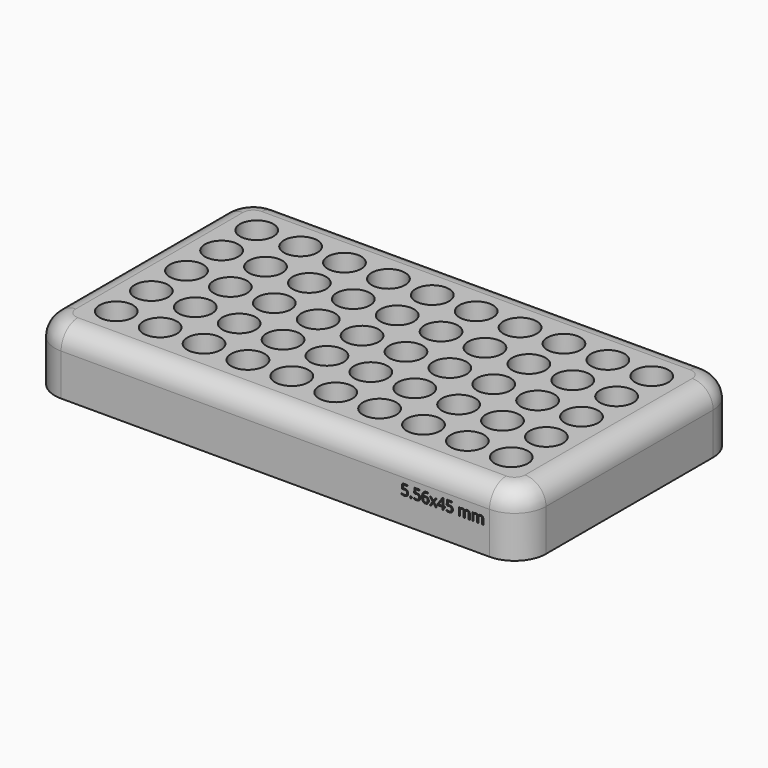
from build123d import *

# Parameters (mm, degrees)
F1_DEPTH     = 19.05
F2_R         = 6.35
F3_R         = 5.08
F4_DEPTH     = 9.525
F5_R         = 3.302
F6_DEPTH     = 15.24
F7_TEXT_SIZE = 4.4154715341
F8_DEPTH     = 1.5875


# Not quite as in the source:
# - Text() gives the source's letters only with a copy of the font that has no kerning and outlines rounded to 1/6400 em; it was checked with that copy


with BuildPart() as f1:
    # F0 (on Top) → F1 (new body)
    with BuildSketch(Plane.XY):
        with BuildLine():
            Line((96.05817945, 87.4035315238), (-34.11682055, 87.4035315238))
            ThreePointArc((-34.11682055, 87.4035315238), (-40.8520126408, 84.6137236146), (-43.64182055, 77.8785315238))
            Line((-43.64182055, 77.8785315238), (-43.64182055, 14.3785315238))
            ThreePointArc((-43.64182055, 14.3785315238), (-40.8520126408, 7.643339433), (-34.11682055, 4.8535315238))
            Line((-34.11682055, 4.8535315238), (96.05817945, 4.8535315238))
            ThreePointArc((96.05817945, 4.8535315238), (102.7933715408, 7.643339433), (105.58317945, 14.3785315238))
            Line((105.58317945, 14.3785315238), (105.58317945, 77.8785315238))
            ThreePointArc((105.58317945, 77.8785315238), (102.7933715408, 84.6137236146), (96.05817945, 87.4035315238))
        make_face()
    extrude(amount=F1_DEPTH)

    # F2
    f2_edges = [f1.edges().sort_by_distance(p)[0] for p in [
        (30.970679, 4.853532, 19.05),
    ]]
    fillet(f2_edges, radius=F2_R)

    # F3 (on face) → F4 (cut)
    with BuildSketch(Plane.XY.offset(19.05)):
        with Locations((-29.03682055, 72.7985315238)):
            Circle(F3_R)
        with Locations((-15.70182055, 72.7985315238)):
            Circle(F3_R)
        with Locations((-2.36682055, 72.7985315238)):
            Circle(F3_R)
        with Locations((10.96817945, 72.7985315238)):
            Circle(F3_R)
        with Locations((24.30317945, 72.7985315238)):
            Circle(F3_R)
        with Locations((37.63817945, 72.7985315238)):
            Circle(F3_R)
        with Locations((64.30817945, 72.7985315238)):
            Circle(F3_R)
        with Locations((50.97317945, 72.7985315238)):
            Circle(F3_R)
        with Locations((90.97817945, 72.7985315238)):
            Circle(F3_R)
        with Locations((77.64317945, 72.7985315238)):
            Circle(F3_R)
        with Locations((-29.03682055, 59.4635315238)):
            Circle(F3_R)
        with Locations((-15.70182055, 59.4635315238)):
            Circle(F3_R)
        with Locations((-2.36682055, 59.4635315238)):
            Circle(F3_R)
        with Locations((10.96817945, 59.4635315238)):
            Circle(F3_R)
        with Locations((24.30317945, 59.4635315238)):
            Circle(F3_R)
        with Locations((37.63817945, 59.4635315238)):
            Circle(F3_R)
        with Locations((50.97317945, 59.4635315238)):
            Circle(F3_R)
        with Locations((64.30817945, 59.4635315238)):
            Circle(F3_R)
        with Locations((77.64317945, 59.4635315238)):
            Circle(F3_R)
        with Locations((90.97817945, 59.4635315238)):
            Circle(F3_R)
        with Locations((90.97817945, 46.1285315238)):
            Circle(F3_R)
        with Locations((77.64317945, 46.1285315238)):
            Circle(F3_R)
        with Locations((64.30817945, 46.1285315238)):
            Circle(F3_R)
        with Locations((50.97317945, 46.1285315238)):
            Circle(F3_R)
        with Locations((37.63817945, 46.1285315238)):
            Circle(F3_R)
        with Locations((24.30317945, 46.1285315238)):
            Circle(F3_R)
        with Locations((10.96817945, 46.1285315238)):
            Circle(F3_R)
        with Locations((-2.36682055, 46.1285315238)):
            Circle(F3_R)
        with Locations((-15.70182055, 46.1285315238)):
            Circle(F3_R)
        with Locations((-29.03682055, 46.1285315238)):
            Circle(F3_R)
        with Locations((-29.03682055, 32.7935315238)):
            Circle(F3_R)
        with Locations((-15.70182055, 32.7935315238)):
            Circle(F3_R)
        with Locations((-2.36682055, 32.7935315238)):
            Circle(F3_R)
        with Locations((10.96817945, 32.7935315238)):
            Circle(F3_R)
        with Locations((24.30317945, 32.7935315238)):
            Circle(F3_R)
        with Locations((37.63817945, 32.7935315238)):
            Circle(F3_R)
        with Locations((50.97317945, 32.7935315238)):
            Circle(F3_R)
        with Locations((64.30817945, 32.7935315238)):
            Circle(F3_R)
        with Locations((77.64317945, 32.7935315238)):
            Circle(F3_R)
        with Locations((90.97817945, 32.7935315238)):
            Circle(F3_R)
        with Locations((90.97817945, 19.4585315238)):
            Circle(F3_R)
        with Locations((77.64317945, 19.4585315238)):
            Circle(F3_R)
        with Locations((64.30817945, 19.4585315238)):
            Circle(F3_R)
        with Locations((50.97317945, 19.4585315238)):
            Circle(F3_R)
        with Locations((37.63817945, 19.4585315238)):
            Circle(F3_R)
        with Locations((24.30317945, 19.4585315238)):
            Circle(F3_R)
        with Locations((10.96817945, 19.4585315238)):
            Circle(F3_R)
        with Locations((-2.36682055, 19.4585315238)):
            Circle(F3_R)
        with Locations((-15.70182055, 19.4585315238)):
            Circle(F3_R)
        with Locations((-29.03682055, 19.4585315238)):
            Circle(F3_R)
    extrude(amount=-F4_DEPTH, mode=Mode.SUBTRACT)

    # F5 (on face) → F6 (cut)
    with BuildSketch(Plane.XY.offset(19.05)):
        with Locations((-29.03682055, 72.7985315238)):
            Circle(F5_R)
        with Locations((-15.70182055, 72.7985315238)):
            Circle(F5_R)
        with Locations((-2.36682055, 72.7985315238)):
            Circle(F5_R)
        with Locations((10.96817945, 72.7985315238)):
            Circle(F5_R)
        with Locations((24.30317945, 72.7985315238)):
            Circle(F5_R)
        with Locations((37.63817945, 72.7985315238)):
            Circle(F5_R)
        with Locations((50.97317945, 72.7985315238)):
            Circle(F5_R)
        with Locations((64.30817945, 72.7985315238)):
            Circle(F5_R)
        with Locations((77.64317945, 72.7985315238)):
            Circle(F5_R)
        with Locations((90.97817945, 72.7985315238)):
            Circle(F5_R)
        with Locations((90.97817945, 59.4635315238)):
            Circle(F5_R)
        with Locations((77.64317945, 59.4635315238)):
            Circle(F5_R)
        with Locations((64.30817945, 59.4635315238)):
            Circle(F5_R)
        with Locations((50.97317945, 59.4635315238)):
            Circle(F5_R)
        with Locations((24.30317945, 59.4635315238)):
            Circle(F5_R)
        with Locations((10.96817945, 59.4635315238)):
            Circle(F5_R)
        with Locations((-2.36682055, 59.4635315238)):
            Circle(F5_R)
        with Locations((-15.70182055, 59.4635315238)):
            Circle(F5_R)
        with Locations((-29.03682055, 59.4635315238)):
            Circle(F5_R)
        with Locations((-29.03682055, 46.1285315238)):
            Circle(F5_R)
        with Locations((-15.70182055, 46.1285315238)):
            Circle(F5_R)
        with Locations((-2.36682055, 46.1285315238)):
            Circle(F5_R)
        with Locations((10.96817945, 46.1285315238)):
            Circle(F5_R)
        with Locations((24.30317945, 46.1285315238)):
            Circle(F5_R)
        with Locations((37.63817945, 46.1285315238)):
            Circle(F5_R)
        with Locations((50.97317945, 46.1285315238)):
            Circle(F5_R)
        with Locations((64.30817945, 46.1285315238)):
            Circle(F5_R)
        with Locations((77.64317945, 46.1285315238)):
            Circle(F5_R)
        with Locations((90.97817945, 46.1285315238)):
            Circle(F5_R)
        with Locations((37.63817945, 59.4635315238)):
            Circle(F5_R)
        with Locations((90.97817945, 32.7935315238)):
            Circle(F5_R)
        with Locations((77.64317945, 32.7935315238)):
            Circle(F5_R)
        with Locations((64.30817945, 32.7935315238)):
            Circle(F5_R)
        with Locations((50.97317945, 32.7935315238)):
            Circle(F5_R)
        with Locations((37.63817945, 32.7935315238)):
            Circle(F5_R)
        with Locations((24.30317945, 32.7935315238)):
            Circle(F5_R)
        with Locations((10.96817945, 32.7935315238)):
            Circle(F5_R)
        with Locations((-2.36682055, 32.7935315238)):
            Circle(F5_R)
        with Locations((-15.70182055, 32.7935315238)):
            Circle(F5_R)
        with Locations((-29.03682055, 32.7935315238)):
            Circle(F5_R)
        with Locations((-29.03682055, 19.4585315238)):
            Circle(F5_R)
        with Locations((-15.70182055, 19.4585315238)):
            Circle(F5_R)
        with Locations((-2.36682055, 19.4585315238)):
            Circle(F5_R)
        with Locations((10.96817945, 19.4585315238)):
            Circle(F5_R)
        with Locations((24.30317945, 19.4585315238)):
            Circle(F5_R)
        with Locations((37.63817945, 19.4585315238)):
            Circle(F5_R)
        with Locations((50.97317945, 19.4585315238)):
            Circle(F5_R)
        with Locations((64.30817945, 19.4585315238)):
            Circle(F5_R)
        with Locations((77.64317945, 19.4585315238)):
            Circle(F5_R)
        with Locations((90.97817945, 19.4585315238)):
            Circle(F5_R)
    extrude(amount=-F6_DEPTH, mode=Mode.SUBTRACT)

    # F7 (on face) → F8 (cut)
    with BuildSketch(Plane.XZ.offset(-4.8535315238)):
        with Locations((69.07067945, 7.9333604954)):
            Text('5.56x45 mm', F7_TEXT_SIZE, font='Open Sans', text_align=(TextAlign.LEFT, TextAlign.BOTTOM))
    extrude(amount=-F8_DEPTH, mode=Mode.SUBTRACT)


solid = f1.part
